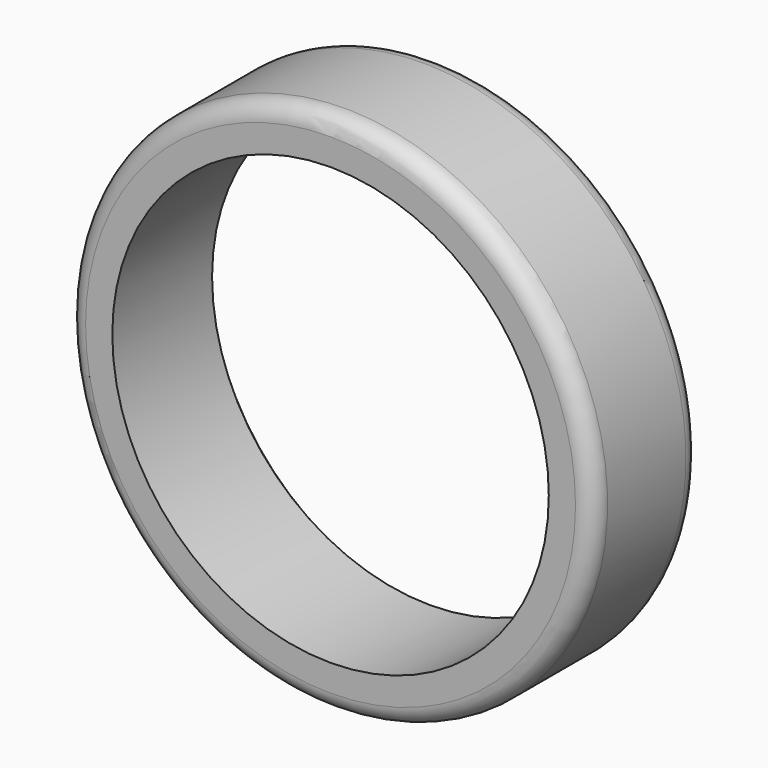
from build123d import *

# Parameters (mm, degrees)
F2_R    = 1.99999
F3_SIZE = 0.99999


# Not quite as in the source:
# - a fillet or chamfer is up to 0.001 mm smaller than in the source, because OpenCascade refuses the exact size


with BuildPart() as f1:
    # F0 (on Top) → F1 (revolve)
    with BuildSketch(Plane.XY):
        Polygon((-24.5, 0), (-24.5, 14.3020306939), (-24.5, 15), (-25.5, 15), (-25.5, 5), (-27.5, 5), (-27.5, 15), (-29.5, 15), (-29.5, 0), align=None)
    revolve(axis=Axis((0, 7.5544440188, 0), (0, -1, 0)))

    # F2 (radius 2 in the source; OpenCascade refuses exactly that, so slightly less here)
    f2_edges = [f1.edges().sort_by_distance(p)[0] for p in [
        (29.5, 15, 0),
        (29.5, 0, 0),
    ]]
    fillet(f2_edges, radius=F2_R)

    # F3 (size 1 in the source; OpenCascade refuses exactly that, so slightly less here)
    f3_edges = [f1.edges().sort_by_distance(p)[0] for p in [
        (24.5, 15, 0),
    ]]
    chamfer(f3_edges, length=F3_SIZE)


solid = f1.part
